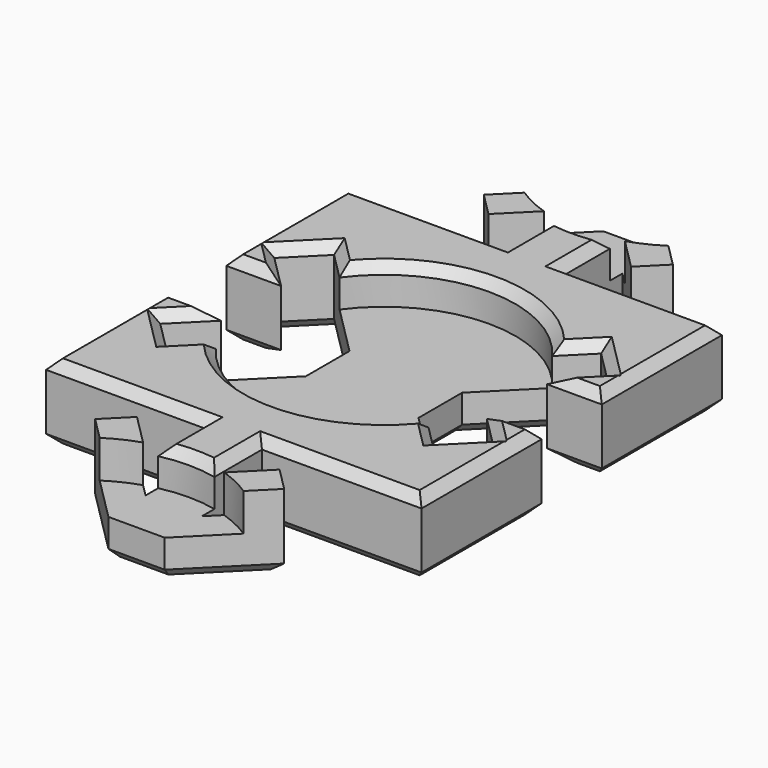
from build123d import *

# Parameters (mm, degrees)
F1_DEPTH      = 4
F4_R          = 7
F5_DEPTH      = 2
F6_T1_DEPTH   = 3.3367062638
F6_T3_DEPTH   = 2.5
F6_T5_DEPTH   = 3.8287347128
F6_T7_DEPTH   = 5.4895762068
F6_T9_DEPTH   = 10.571682988
F6_T11_DEPTH  = 9.785841494
F6_T13_DEPTH  = 4.4484443284
F6_T15_DEPTH  = 9.785841494
F6_T17_DEPTH  = 5.4895762068
F6_T19_DEPTH  = 3.8287347128
F6_T21_DEPTH  = 2.5
F6_T23_DEPTH  = 3.3367062638
F6_T25_DEPTH  = 4.4484443284
F6_T27_DEPTH  = 10.571682988
F6_T29_DEPTH  = 3.8287347128
F6_T31_DEPTH  = 2.5
F6_T33_DEPTH  = 3.3367062638
F6_T35_DEPTH  = 3.3367062638
F6_T37_DEPTH  = 2.5
F6_T39_DEPTH  = 3.8287347128
F6_T41_DEPTH  = 4.321682988
F6_T43_DEPTH  = 4.321682988
F6_T45_DEPTH  = 7.571682988
F6_T47_DEPTH  = 5.571682988
F6_T49_DEPTH  = 7.571682988
F6_T51_DEPTH  = 4.321682988
F6_T53_DEPTH  = 4.321682988
F6_T55_DEPTH  = 7.571682988
F6_T57_DEPTH  = 7.571682988
F6_T60_ANGLE  = 129.037666836
F6_T64_ANGLE  = 45.7974010276
F6_T70_ANGLE  = 45.7974010276
F6_T74_ANGLE  = 129.037666836
F6_T78_DEPTH  = 5.821682988
F6_T83_DEPTH  = 5.285841494
F6_T88_DEPTH  = 7.1017054858
F6_T93_DEPTH  = 5.4785372375
F6_T99_DEPTH  = 7.1017054858
F6_T104_DEPTH = 5.285841494
F6_T109_DEPTH = 5.821682988
F6_T114_DEPTH = 5.821682988
F6_T119_DEPTH = 5.285841494
F6_T124_DEPTH = 7.1017054858
F6_T129_DEPTH = 5.4785372375
F6_T135_DEPTH = 7.1017054858
F6_T140_DEPTH = 5.285841494
F6_T145_DEPTH = 5.821682988
F6_T151_DEPTH = 3.785841494
F6_T155_DEPTH = 4.6225477578
F6_T162_DEPTH = 5.1145762068
F6_T167_DEPTH = 3.785841494
F6_T175_DEPTH = 5.7342858224
F6_T179_DEPTH = 9.785841494
F6_T186_DEPTH = 9.785841494
F6_T190_DEPTH = 5.7342858224
F6_T197_DEPTH = 3.785841494
F6_T202_DEPTH = 5.1145762068
F6_T210_DEPTH = 4.6225477578
F6_T214_DEPTH = 3.785841494
F6_T221_DEPTH = 9.785841494
F6_T225_DEPTH = 5.7342858224
F6_T232_DEPTH = 3.785841494
F6_T237_DEPTH = 5.1145762068
F6_T245_DEPTH = 4.6225477578
F6_T249_DEPTH = 3.785841494
F6_T256_DEPTH = 3.785841494
F6_T260_DEPTH = 4.6225477578
F6_T267_DEPTH = 5.1145762068
F6_T272_DEPTH = 3.785841494
F6_T280_DEPTH = 5.7342858224
F6_T284_DEPTH = 9.785841494
F6_T291_DEPTH = 4.535841494
F6_T295_DEPTH = 5.285841494
F6_T302_DEPTH = 6.571682988
F6_T306_DEPTH = 9.785841494
F6_T313_DEPTH = 5.1145762068
F6_T318_DEPTH = 3.785841494
F6_T326_DEPTH = 3.785841494
F6_T330_DEPTH = 8.3875469798
F6_T337_DEPTH = 7.1017054858
F6_T341_DEPTH = 5.4785372375
F6_T348_DEPTH = 5.4785372375
F6_T352_DEPTH = 7.1017054858
F6_T359_DEPTH = 8.3875469798
F6_T363_DEPTH = 3.785841494
F6_T370_DEPTH = 3.785841494
F6_T375_DEPTH = 5.1145762068
F6_T383_DEPTH = 9.785841494
F6_T387_DEPTH = 6.571682988
F6_T394_DEPTH = 5.285841494
F6_T398_DEPTH = 4.535841494
F6_T405_DEPTH = 4.535841494
F6_T409_DEPTH = 5.285841494
F6_T416_DEPTH = 6.571682988
F6_T420_DEPTH = 9.785841494
F6_T427_DEPTH = 5.1145762068
F6_T432_DEPTH = 3.785841494
F6_T440_DEPTH = 3.785841494
F6_T444_DEPTH = 8.3875469798
F6_T451_DEPTH = 7.1017054858
F6_T455_DEPTH = 5.4785372375
F6_T462_DEPTH = 5.4785372375
F6_T466_DEPTH = 7.1017054858
F6_T473_DEPTH = 8.3875469798
F6_T477_DEPTH = 3.785841494
F6_T484_DEPTH = 3.785841494
F6_T489_DEPTH = 5.1145762068
F6_T497_DEPTH = 9.785841494
F6_T501_DEPTH = 6.571682988
F6_T508_DEPTH = 5.285841494
F6_T512_DEPTH = 4.535841494


# Not quite as in the source:
# - a fillet or chamfer that OpenCascade refuses, or shapes differently, is made with other operations: its cross-section is extruded or revolved along the edge and cut away or added


with BuildPart() as f1:
    # F0 (on Top) → F1 (new body)
    with BuildSketch(Plane.XY):
        Polygon((-1.5, 10), (0, 10), (0, 16.4748737342), (-1.5, 16.4748737342), (-5.0355339059, 12.9393398282), (-3.7980970389, 11.7019029611), (-1.5, 14), align=None)
        Polygon((-3, 0), (0, 0), (0, 10), (-1.5, 10), (-10, 10), (-10, 2), (-7.0821067812, 2), (-8.88020382, 3.7980970389), (-7.1124368671, 5.5658639918), (-3, 1.4534271247), align=None)
    extrude(amount=F1_DEPTH)

    # F2: F1 across plane


with BuildPart() as f1_1:
    add(f1.part)
    add(f1.part.mirror(Plane.YZ))

    # F3: F1 across plane


with BuildPart() as f1_2:
    add(f1_1.part)
    add(f1_1.part.mirror(Plane.XZ))

    # F4 (on face) → F5 (cut)
    with BuildSketch(Plane.XY.offset(4)):
        Circle(F4_R)
        with Locations((0, 20)):
            Circle(F4_R)
        with Locations((0, -20)):
            Circle(F4_R)
    extrude(amount=-F5_DEPTH, mode=Mode.SUBTRACT)

    # F6: chamfer of 0.5 on 76 edges, made by hand

    # F6_s2 → F6_t1 (cut)
    with BuildSketch(Plane(origin=(6.3391504294, -6.3391504294, 0), x_dir=(0, 0, 1), z_dir=(-0.7071067812, 0.7071067812, 0))):
        Polygon((3.5, 1.0935921677), (4, 0.5935921677), (4, 1.0935921677), align=None)
    extrude(amount=F6_T1_DEPTH, mode=Mode.SUBTRACT)

    # F6_s4 → F6_t3 (cut)
    with BuildSketch(Plane(origin=(2.5410533906, 2.5410533906, 0), x_dir=(0, 0, 1), z_dir=(-0.7071067812, -0.7071067812, 0))):
        Polygon((3.5, -8.9649125113), (4, -9.4649125113), (4, -8.9649125113), align=None)
        Polygon((0, -9.4649125113), (0.5, -8.9649125113), (0, -8.9649125113), align=None)
    extrude(amount=F6_T3_DEPTH, mode=Mode.SUBTRACT)

    # F6_s6 → F6_t5 (cut)
    with BuildSketch(Plane(origin=(3.6318261507, -3.6318261507, 0), x_dir=(0, 0, 1), z_dir=(0.7071067812, -0.7071067812, 0))):
        Polygon((3.5, -3.5935921677), (4, -4.0935921677), (4, -3.5935921677), align=None)
        Polygon((0, -4.0935921677), (0.5, -3.5935921677), (0, -3.5935921677), align=None)
    extrude(amount=F6_T5_DEPTH, mode=Mode.SUBTRACT)

    # F6_s8 → F6_t7 (cut)
    with BuildSketch(Plane.YZ.offset(5.7962652872)):
        Polygon((-2, 3.5), (-2.5, 4), (-2, 4), align=None)
        Polygon((2, 3.5), (2.5, 4), (2, 4), align=None)
        Polygon((-2.5, 0), (-2, 0.5), (-2, 0), align=None)
        Polygon((2.5, 0), (2, 0.5), (2, 0), align=None)
    extrude(amount=F6_T7_DEPTH, mode=Mode.SUBTRACT)

    # F6_s10 → F6_t9 (cut)
    with BuildSketch(Plane.XZ.offset(0.714158506)):
        Polygon((10, 3.5), (9.5, 4), (10, 4), align=None)
        Polygon((-10, 3.5), (-9.5, 4), (-10, 4), align=None)
        Polygon((-9.5, 0), (-10, 0.5), (-10, 0), align=None)
        Polygon((9.5, 0), (10, 0.5), (10, 0), align=None)
    extrude(amount=F6_T9_DEPTH, mode=Mode.SUBTRACT)

    # F6_s12 → F6_t11 (cut)
    with BuildSketch(Plane.YZ.offset(1.5)):
        Polygon((-10, 3.5), (-9.5, 4), (-10, 4), align=None)
        Polygon((10, 3.5), (9.5, 4), (10, 4), align=None)
        Polygon((-9.5, 0), (-10, 0.5), (-10, 0), align=None)
        Polygon((9.5, 0), (10, 0.5), (10, 0), align=None)
    extrude(amount=F6_T11_DEPTH, mode=Mode.SUBTRACT)

    # F6_s14 → F6_t13 (cut)
    with BuildSketch(Plane.XZ.offset(10)):
        Polygon((1.5, 3.5), (1, 4), (1.5, 4), align=None)
        Polygon((-1.5, 3.5), (-1, 4), (-1.5, 4), align=None)
    extrude(amount=F6_T13_DEPTH, mode=Mode.SUBTRACT)

    # F6_s16 → F6_t15 (cut)
    with BuildSketch(Plane.YZ.offset(-11.285841494)):
        Polygon((-10, 3.5), (-9.5, 4), (-10, 4), align=None)
        Polygon((10, 3.5), (9.5, 4), (10, 4), align=None)
        Polygon((9.5, 0), (10, 0.5), (10, 0), align=None)
        Polygon((-9.5, 0), (-10, 0.5), (-10, 0), align=None)
    extrude(amount=F6_T15_DEPTH, mode=Mode.SUBTRACT)

    # F6_s18 → F6_t17 (cut)
    with BuildSketch(Plane.YZ.offset(-11.285841494)):
        Polygon((-2, 3.5), (-2.5, 4), (-2, 4), align=None)
        Polygon((2, 3.5), (2.5, 4), (2, 4), align=None)
        Polygon((2.5, 0), (2, 0.5), (2, 0), align=None)
        Polygon((-2.5, 0), (-2, 0.5), (-2, 0), align=None)
    extrude(amount=F6_T17_DEPTH, mode=Mode.SUBTRACT)

    # F6_s20 → F6_t19 (cut)
    with BuildSketch(Plane(origin=(-3.6318261507, -3.6318261507, 0), x_dir=(0, 0, 1), z_dir=(-0.7071067812, -0.7071067812, 0))):
        Polygon((3.5, 3.5935921677), (4, 4.0935921677), (4, 3.5935921677), align=None)
        Polygon((0, 4.0935921677), (0.5, 3.5935921677), (0, 3.5935921677), align=None)
    extrude(amount=F6_T19_DEPTH, mode=Mode.SUBTRACT)

    # F6_s22 → F6_t21 (cut)
    with BuildSketch(Plane(origin=(-2.5410533906, 2.5410533906, 0), x_dir=(0, 0, 1), z_dir=(0.7071067812, -0.7071067812, 0))):
        Polygon((3.5, 8.9649125113), (4, 9.4649125113), (4, 8.9649125113), align=None)
        Polygon((0, 9.4649125113), (0.5, 8.9649125113), (0, 8.9649125113), align=None)
    extrude(amount=F6_T21_DEPTH, mode=Mode.SUBTRACT)

    # F6_s24 → F6_t23 (cut)
    with BuildSketch(Plane(origin=(-6.3391504294, -6.3391504294, 0), x_dir=(0, 0, 1), z_dir=(0.7071067812, 0.7071067812, 0))):
        Polygon((3.5, -1.0935921677), (4, -0.5935921677), (4, -1.0935921677), align=None)
    extrude(amount=F6_T23_DEPTH, mode=Mode.SUBTRACT)

    # F6_s26 → F6_t25 (cut)
    with BuildSketch(Plane.XZ.offset(-14.4484443284)):
        Polygon((1.5, 3.5), (1, 4), (1.5, 4), align=None)
        Polygon((-1.5, 3.5), (-1, 4), (-1.5, 4), align=None)
    extrude(amount=F6_T25_DEPTH, mode=Mode.SUBTRACT)

    # F6_s28 → F6_t27 (cut)
    with BuildSketch(Plane.XZ.offset(-11.285841494)):
        Polygon((10, 3.5), (9.5, 4), (10, 4), align=None)
        Polygon((-10, 3.5), (-9.5, 4), (-10, 4), align=None)
        Polygon((-9.5, 0), (-10, 0.5), (-10, 0), align=None)
        Polygon((9.5, 0), (10, 0.5), (10, 0), align=None)
    extrude(amount=F6_T27_DEPTH, mode=Mode.SUBTRACT)

    # F6_s30 → F6_t29 (cut)
    with BuildSketch(Plane(origin=(3.6318261507, 3.6318261507, 0), x_dir=(0, 0, 1), z_dir=(0.7071067812, 0.7071067812, 0))):
        Polygon((3.5, 3.5935921677), (4, 4.0935921677), (4, 3.5935921677), align=None)
        Polygon((0, 4.0935921677), (0.5, 3.5935921677), (0, 3.5935921677), align=None)
    extrude(amount=F6_T29_DEPTH, mode=Mode.SUBTRACT)

    # F6_s32 → F6_t31 (cut)
    with BuildSketch(Plane(origin=(2.5410533906, -2.5410533906, 0), x_dir=(0, 0, 1), z_dir=(-0.7071067812, 0.7071067812, 0))):
        Polygon((3.5, 8.9649125113), (4, 9.4649125113), (4, 8.9649125113), align=None)
        Polygon((0, 9.4649125113), (0.5, 8.9649125113), (0, 8.9649125113), align=None)
    extrude(amount=F6_T31_DEPTH, mode=Mode.SUBTRACT)

    # F6_s34 → F6_t33 (cut)
    with BuildSketch(Plane(origin=(6.3391504294, 6.3391504294, 0), x_dir=(0, 0, 1), z_dir=(-0.7071067812, -0.7071067812, 0))):
        Polygon((3.5, -1.0935921677), (4, -0.5935921677), (4, -1.0935921677), align=None)
    extrude(amount=F6_T33_DEPTH, mode=Mode.SUBTRACT)

    # F6_s36 → F6_t35 (cut)
    with BuildSketch(Plane(origin=(-6.3391504294, 6.3391504294, 0), x_dir=(0, 0, 1), z_dir=(0.7071067812, -0.7071067812, 0))):
        Polygon((3.5, 1.0935921677), (4, 0.5935921677), (4, 1.0935921677), align=None)
    extrude(amount=F6_T35_DEPTH, mode=Mode.SUBTRACT)

    # F6_s38 → F6_t37 (cut)
    with BuildSketch(Plane(origin=(-2.5410533906, -2.5410533906, 0), x_dir=(0, 0, 1), z_dir=(0.7071067812, 0.7071067812, 0))):
        Polygon((3.5, -8.9649125113), (4, -9.4649125113), (4, -8.9649125113), align=None)
        Polygon((0, -9.4649125113), (0.5, -8.9649125113), (0, -8.9649125113), align=None)
    extrude(amount=F6_T37_DEPTH, mode=Mode.SUBTRACT)

    # F6_s40 → F6_t39 (cut)
    with BuildSketch(Plane(origin=(-3.6318261507, 3.6318261507, 0), x_dir=(0, 0, 1), z_dir=(-0.7071067812, 0.7071067812, 0))):
        Polygon((3.5, -3.5935921677), (4, -4.0935921677), (4, -3.5935921677), align=None)
        Polygon((0, -4.0935921677), (0.5, -3.5935921677), (0, -3.5935921677), align=None)
    extrude(amount=F6_T39_DEPTH, mode=Mode.SUBTRACT)

    # F6_s42 → F6_t41 (cut)
    with BuildSketch(Plane(origin=(-9.896664107, 9.896664107, 0), x_dir=(0, 0, 1), z_dir=(0.7071067812, -0.7071067812, 0))):
        Polygon((0.5, -5.5888347648), (0, -6.0888347648), (0, -5.5888347648), align=None)
    extrude(amount=F6_T41_DEPTH, mode=Mode.SUBTRACT)

    # F6_s44 → F6_t43 (cut)
    with BuildSketch(Plane(origin=(-9.896664107, -9.896664107, 0), x_dir=(0, 0, 1), z_dir=(0.7071067812, 0.7071067812, 0))):
        Polygon((0, 6.0888347648), (0.5, 5.5888347648), (0, 5.5888347648), align=None)
    extrude(amount=F6_T43_DEPTH, mode=Mode.SUBTRACT)

    # F6_s46 → F6_t45 (cut)
    with BuildSketch(Plane(origin=(8.396664107, -8.396664107, 0), x_dir=(0, 0, 1), z_dir=(-0.7071067812, 0.7071067812, 0))):
        Polygon((0, -12.2101551084), (0.5, -12.7101551084), (0, -12.7101551084), align=None)
    extrude(amount=F6_T45_DEPTH, mode=Mode.SUBTRACT)

    # F6_s48 → F6_t47 (cut)
    with BuildSketch(Plane.YZ.offset(-2.785841494)):
        Polygon((-15.9748737342, 0), (-16.4748737342, 0.5), (-16.4748737342, 0), align=None)
        Polygon((15.9748737342, 0), (16.4748737342, 0.5), (16.4748737342, 0), align=None)
    extrude(amount=F6_T47_DEPTH, mode=Mode.SUBTRACT)

    # F6_s50 → F6_t49 (cut)
    with BuildSketch(Plane(origin=(-8.396664107, -8.396664107, 0), x_dir=(0, 0, 1), z_dir=(0.7071067812, 0.7071067812, 0))):
        Polygon((0, 12.2101551084), (0.5, 12.7101551084), (0, 12.7101551084), align=None)
    extrude(amount=F6_T49_DEPTH, mode=Mode.SUBTRACT)

    # F6_s52 → F6_t51 (cut)
    with BuildSketch(Plane(origin=(9.896664107, -9.896664107, 0), x_dir=(0, 0, 1), z_dir=(-0.7071067812, 0.7071067812, 0))):
        Polygon((0, -6.0888347648), (0.5, -5.5888347648), (0, -5.5888347648), align=None)
    extrude(amount=F6_T51_DEPTH, mode=Mode.SUBTRACT)

    # F6_s54 → F6_t53 (cut)
    with BuildSketch(Plane(origin=(9.896664107, 9.896664107, 0), x_dir=(0, 0, 1), z_dir=(-0.7071067812, -0.7071067812, 0))):
        Polygon((0, 6.0888347648), (0.5, 5.5888347648), (0, 5.5888347648), align=None)
    extrude(amount=F6_T53_DEPTH, mode=Mode.SUBTRACT)

    # F6_s56 → F6_t55 (cut)
    with BuildSketch(Plane(origin=(-8.396664107, 8.396664107, 0), x_dir=(0, 0, 1), z_dir=(0.7071067812, -0.7071067812, 0))):
        Polygon((0, -12.2101551084), (0.5, -12.7101551084), (0, -12.7101551084), align=None)
    extrude(amount=F6_T55_DEPTH, mode=Mode.SUBTRACT)

    # F6_s58 → F6_t57 (cut)
    with BuildSketch(Plane(origin=(8.396664107, 8.396664107, 0), x_dir=(0, 0, 1), z_dir=(-0.7071067812, -0.7071067812, 0))):
        Polygon((0.5, 12.7101551084), (0, 12.2101551084), (0, 12.7101551084), align=None)
    extrude(amount=F6_T57_DEPTH, mode=Mode.SUBTRACT)

    # F6_s59 → F6_t60 (revolve, cut)
    with BuildSketch(Plane(origin=(0, 0, 0), x_dir=(0, 0, 1), z_dir=(-0.4302143891, 0.9027267468, 0))):
        Polygon((3.5, -7), (4, -7.5), (4, -7), align=None)
    revolve(axis=Axis((0, 0, 4), (0, 0, 1)), revolution_arc=F6_T60_ANGLE, mode=Mode.SUBTRACT)


with BuildPart() as f6_tool62:
    # F6_s63 → F6_t64 (revolve)
    with BuildSketch(Plane(origin=(7.1687898307, -3.0280237835, 0), x_dir=(0, 0, 1), z_dir=(0.9211942308, -0.3891030573, 0))):
        Polygon((4, 10.9238846156), (3.5, 11.4238846156), (4, 11.4238846156), align=None)
    revolve(axis=Axis((0, -20, 4), (0, 0, 1)), revolution_arc=F6_T64_ANGLE)

    split(bisect_by=Plane(origin=(-7.75, -7.75, 0), x_dir=(0, 0, 1), z_dir=(0.7071067812, 0.7071067812, 0)), keep=Keep.TOP)

    split(bisect_by=Plane.YZ.offset(1.5), keep=Keep.BOTTOM)


with BuildPart() as f1_3:
    add(f1_2.part)

    # F6_t61: cut F6_tool62
    add(f6_tool62.part, mode=Mode.SUBTRACT)


with BuildPart() as f6_tool68:
    # F6_s69 → F6_t70 (revolve)
    with BuildSketch(Plane(origin=(-7.1687898307, 3.0280237835, 0), x_dir=(0, 0, 1), z_dir=(-0.9211942308, 0.3891030573, 0))):
        Polygon((3.5, 11.4238846156), (4, 10.9238846156), (4, 11.4238846156), align=None)
    revolve(axis=Axis((0, 20, 4), (0, 0, 1)), revolution_arc=F6_T70_ANGLE)

    split(bisect_by=Plane.YZ.offset(-1.5), keep=Keep.TOP)

    split(bisect_by=Plane(origin=(7.75, 7.75, 0), x_dir=(0, 0, 1), z_dir=(-0.7071067812, -0.7071067812, 0)), keep=Keep.TOP)


with BuildPart() as f1_4:
    add(f1_3.part)

    # F6_t67: cut F6_tool68
    add(f6_tool68.part, mode=Mode.SUBTRACT)

    # F6_s73 → F6_t74 (revolve, cut)
    with BuildSketch(Plane(origin=(0, 0, 0), x_dir=(0, 0, 1), z_dir=(0.4302143891, -0.9027267468, 0))):
        Polygon((4, -7.5), (3.5, -7), (4, -7), align=None)
    revolve(axis=Axis((0, 0, 4), (0, 0, 1)), revolution_arc=F6_T74_ANGLE, mode=Mode.SUBTRACT)


with BuildPart() as f6_tool76:
    # F6_s77 → F6_t78 (new body)
    with BuildSketch(Plane(origin=(3.0426757212, 3.0426757212, 0), x_dir=(0, 0, 1), z_dir=(0.7071067812, 0.7071067812, 0))):
        Polygon((0.5, -10.9601551084), (0, -11.4601551084), (0, -10.9601551084), align=None)
    extrude(amount=F6_T78_DEPTH)

    split(bisect_by=Plane.YZ.offset(-1.5), keep=Keep.BOTTOM)


with BuildPart() as f1_5:
    add(f1_4.part)

    # F6_t75: cut F6_tool76
    add(f6_tool76.part, mode=Mode.SUBTRACT)


with BuildPart() as f6_tool81:
    # F6_s82 → F6_t83 (new body)
    with BuildSketch(Plane.XZ.offset(-15.285841494)):
        Polygon((-1, 0), (-1.5, 0.5), (-1.5, 0), align=None)
    extrude(amount=F6_T83_DEPTH)

    split(bisect_by=Plane(origin=(-7.75, 7.75, 0), x_dir=(0, 0, 1), z_dir=(0.7071067812, -0.7071067812, 0)), keep=Keep.TOP)


with BuildPart() as f1_6:
    add(f1_5.part)

    # F6_t80: cut F6_tool81
    add(f6_tool81.part, mode=Mode.SUBTRACT)


with BuildPart() as f6_tool86:
    # F6_s87 → F6_t88 (new body)
    with BuildSketch(Plane(origin=(-6.3391504294, 6.3391504294, 0), x_dir=(0, 0, 1), z_dir=(0.7071067812, -0.7071067812, 0))):
        Polygon((0, 0.5935921677), (0.5, 1.0935921677), (0, 1.0935921677), align=None)
    extrude(amount=F6_T88_DEPTH)

    split(bisect_by=Plane.YZ.offset(-3), keep=Keep.BOTTOM)


with BuildPart() as f1_7:
    add(f1_6.part)

    # F6_t85: cut F6_tool86
    add(f6_tool86.part, mode=Mode.SUBTRACT)


with BuildPart() as f6_tool91:
    # F6_s92 → F6_t93 (new body)
    with BuildSketch(Plane.XZ.offset(2.7392686187)):
        Polygon((-2.5, 0), (-3, 0.5), (-3, 0), align=None)
    extrude(amount=-F6_T93_DEPTH)

    split(bisect_by=Plane(origin=(-0.7732864376, -0.7732864376, 0), x_dir=(0, 0, 1), z_dir=(-0.7071067812, -0.7071067812, 0)), keep=Keep.TOP)

    split(bisect_by=Plane(origin=(-0.7732864376, 0.7732864376, 0), x_dir=(0, 0, 1), z_dir=(-0.7071067812, 0.7071067812, 0)), keep=Keep.TOP)


with BuildPart() as f1_8:
    add(f1_7.part)

    # F6_t90: cut F6_tool91
    add(f6_tool91.part, mode=Mode.SUBTRACT)


with BuildPart() as f6_tool97:
    # F6_s98 → F6_t99 (new body)
    with BuildSketch(Plane(origin=(-6.3391504294, -6.3391504294, 0), x_dir=(0, 0, 1), z_dir=(0.7071067812, 0.7071067812, 0))):
        Polygon((0, -0.5935921677), (0.5, -1.0935921677), (0, -1.0935921677), align=None)
    extrude(amount=F6_T99_DEPTH)

    split(bisect_by=Plane.YZ.offset(-3), keep=Keep.BOTTOM)


with BuildPart() as f1_9:
    add(f1_8.part)

    # F6_t96: cut F6_tool97
    add(f6_tool97.part, mode=Mode.SUBTRACT)


with BuildPart() as f6_tool102:
    # F6_s103 → F6_t104 (new body)
    with BuildSketch(Plane.XZ.offset(15.285841494)):
        Polygon((-1, 0), (-1.5, 0.5), (-1.5, 0), align=None)
    extrude(amount=-F6_T104_DEPTH)

    split(bisect_by=Plane(origin=(-7.75, -7.75, 0), x_dir=(0, 0, 1), z_dir=(0.7071067812, 0.7071067812, 0)), keep=Keep.TOP)


with BuildPart() as f1_10:
    add(f1_9.part)

    # F6_t101: cut F6_tool102
    add(f6_tool102.part, mode=Mode.SUBTRACT)


with BuildPart() as f6_tool107:
    # F6_s108 → F6_t109 (new body)
    with BuildSketch(Plane(origin=(3.0426757212, -3.0426757212, 0), x_dir=(0, 0, 1), z_dir=(0.7071067812, -0.7071067812, 0))):
        Polygon((0, 11.4601551084), (0.5, 10.9601551084), (0, 10.9601551084), align=None)
    extrude(amount=F6_T109_DEPTH)

    split(bisect_by=Plane.YZ.offset(-1.5), keep=Keep.BOTTOM)


with BuildPart() as f1_11:
    add(f1_10.part)

    # F6_t106: cut F6_tool107
    add(f6_tool107.part, mode=Mode.SUBTRACT)


with BuildPart() as f6_tool112:
    # F6_s113 → F6_t114 (new body)
    with BuildSketch(Plane(origin=(-3.0426757212, -3.0426757212, 0), x_dir=(0, 0, 1), z_dir=(-0.7071067812, -0.7071067812, 0))):
        Polygon((0, -11.4601551084), (0.5, -10.9601551084), (0, -10.9601551084), align=None)
    extrude(amount=F6_T114_DEPTH)

    split(bisect_by=Plane.YZ.offset(1.5), keep=Keep.TOP)


with BuildPart() as f1_12:
    add(f1_11.part)

    # F6_t111: cut F6_tool112
    add(f6_tool112.part, mode=Mode.SUBTRACT)


with BuildPart() as f6_tool117:
    # F6_s118 → F6_t119 (new body)
    with BuildSketch(Plane.XZ.offset(15.285841494)):
        Polygon((1, 0), (1.5, 0.5), (1.5, 0), align=None)
    extrude(amount=-F6_T119_DEPTH)

    split(bisect_by=Plane(origin=(7.75, -7.75, 0), x_dir=(0, 0, 1), z_dir=(-0.7071067812, 0.7071067812, 0)), keep=Keep.TOP)


with BuildPart() as f1_13:
    add(f1_12.part)

    # F6_t116: cut F6_tool117
    add(f6_tool117.part, mode=Mode.SUBTRACT)


with BuildPart() as f6_tool122:
    # F6_s123 → F6_t124 (new body)
    with BuildSketch(Plane(origin=(6.3391504294, -6.3391504294, 0), x_dir=(0, 0, 1), z_dir=(-0.7071067812, 0.7071067812, 0))):
        Polygon((0, 0.5935921677), (0.5, 1.0935921677), (0, 1.0935921677), align=None)
    extrude(amount=F6_T124_DEPTH)

    split(bisect_by=Plane.YZ.offset(3), keep=Keep.TOP)


with BuildPart() as f1_14:
    add(f1_13.part)

    # F6_t121: cut F6_tool122
    add(f6_tool122.part, mode=Mode.SUBTRACT)


with BuildPart() as f6_tool127:
    # F6_s128 → F6_t129 (new body)
    with BuildSketch(Plane.XZ.offset(-2.7392686187)):
        Polygon((2.5, 0), (3, 0.5), (3, 0), align=None)
    extrude(amount=F6_T129_DEPTH)

    split(bisect_by=Plane(origin=(0.7732864376, 0.7732864376, 0), x_dir=(0, 0, 1), z_dir=(0.7071067812, 0.7071067812, 0)), keep=Keep.TOP)

    split(bisect_by=Plane(origin=(0.7732864376, -0.7732864376, 0), x_dir=(0, 0, 1), z_dir=(0.7071067812, -0.7071067812, 0)), keep=Keep.TOP)


with BuildPart() as f1_15:
    add(f1_14.part)

    # F6_t126: cut F6_tool127
    add(f6_tool127.part, mode=Mode.SUBTRACT)


with BuildPart() as f6_tool133:
    # F6_s134 → F6_t135 (new body)
    with BuildSketch(Plane(origin=(6.3391504294, 6.3391504294, 0), x_dir=(0, 0, 1), z_dir=(-0.7071067812, -0.7071067812, 0))):
        Polygon((0, -0.5935921677), (0.5, -1.0935921677), (0, -1.0935921677), align=None)
    extrude(amount=F6_T135_DEPTH)

    split(bisect_by=Plane.YZ.offset(3), keep=Keep.TOP)


with BuildPart() as f1_16:
    add(f1_15.part)

    # F6_t132: cut F6_tool133
    add(f6_tool133.part, mode=Mode.SUBTRACT)


with BuildPart() as f6_tool138:
    # F6_s139 → F6_t140 (new body)
    with BuildSketch(Plane.XZ.offset(-15.285841494)):
        Polygon((1, 0), (1.5, 0.5), (1.5, 0), align=None)
    extrude(amount=F6_T140_DEPTH)

    split(bisect_by=Plane(origin=(7.75, 7.75, 0), x_dir=(0, 0, 1), z_dir=(-0.7071067812, -0.7071067812, 0)), keep=Keep.TOP)


with BuildPart() as f1_17:
    add(f1_16.part)

    # F6_t137: cut F6_tool138
    add(f6_tool138.part, mode=Mode.SUBTRACT)


with BuildPart() as f6_tool143:
    # F6_s144 → F6_t145 (new body)
    with BuildSketch(Plane(origin=(-3.0426757212, 3.0426757212, 0), x_dir=(0, 0, 1), z_dir=(-0.7071067812, 0.7071067812, 0))):
        Polygon((0, 11.4601551084), (0.5, 10.9601551084), (0, 10.9601551084), align=None)
    extrude(amount=F6_T145_DEPTH)

    split(bisect_by=Plane.YZ.offset(1.5), keep=Keep.TOP)


with BuildPart() as f1_18:
    add(f1_17.part)

    # F6_t142: cut F6_tool143
    add(f6_tool143.part, mode=Mode.SUBTRACT)


with BuildPart() as f6_tool149:
    # F6_s150 → F6_t151 (new body)
    with BuildSketch(Plane(origin=(2.5410533906, 2.5410533906, 0), x_dir=(0, 0, 1), z_dir=(-0.7071067812, -0.7071067812, 0))):
        Polygon((3.5, -8.9649125113), (4, -9.4649125113), (4, -8.9649125113), align=None)
    extrude(amount=F6_T151_DEPTH)

    split(bisect_by=Plane(origin=(0.7732864376, 0.7732864376, 0), x_dir=(0, 0, 1), z_dir=(-0.7071067812, -0.7071067812, 0)), keep=Keep.TOP)


with BuildPart() as f6_tool153:
    # F6_s154 → F6_t155 (new body)
    with BuildSketch(Plane(origin=(7.2483776694, -7.2483776694, 0), x_dir=(0, 0, 1), z_dir=(-0.7071067812, 0.7071067812, 0))):
        Polygon((3.5, 1.0935921677), (4, 0.5935921677), (4, 1.0935921677), align=None)
    extrude(amount=F6_T155_DEPTH)

    split(bisect_by=Plane(origin=(6.3391504294, -6.3391504294, 0), x_dir=(0, 0, 1), z_dir=(0.7071067812, -0.7071067812, 0)), keep=Keep.TOP)


with BuildPart() as f6_tool149_1:
    add(f6_tool149.part)

    # F6_t157: intersect F6_tool153
    add(f6_tool153.part, mode=Mode.INTERSECT)


with BuildPart() as f1_19:
    add(f1_18.part)

    # F6_t147: cut F6_tool149
    add(f6_tool149_1.part, mode=Mode.SUBTRACT)


with BuildPart() as f6_tool160:
    # F6_s161 → F6_t162 (new body)
    with BuildSketch(Plane(origin=(3.6318261507, -3.6318261507, 0), x_dir=(0, 0, 1), z_dir=(0.7071067812, -0.7071067812, 0))):
        Polygon((3.5, -3.5935921677), (4, -4.0935921677), (4, -3.5935921677), align=None)
    extrude(amount=F6_T162_DEPTH)

    split(bisect_by=Plane.YZ.offset(10), keep=Keep.BOTTOM)

    split(bisect_by=Plane(origin=(6.3391504294, -6.3391504294, 0), x_dir=(0, 0, 1), z_dir=(0.7071067812, -0.7071067812, 0)), keep=Keep.TOP)


with BuildPart() as f6_tool165:
    # F6_s166 → F6_t167 (new body)
    with BuildSketch(Plane(origin=(3.4502806305, 3.4502806305, 0), x_dir=(0, 0, 1), z_dir=(-0.7071067812, -0.7071067812, 0))):
        Polygon((3.5, -8.9649125113), (4, -9.4649125113), (4, -8.9649125113), align=None)
    extrude(amount=F6_T167_DEPTH)

    split(bisect_by=Plane.YZ.offset(10), keep=Keep.BOTTOM)

    split(bisect_by=Plane(origin=(2.5410533906, 2.5410533906, 0), x_dir=(0, 0, 1), z_dir=(0.7071067812, 0.7071067812, 0)), keep=Keep.TOP)


with BuildPart() as f6_tool160_1:
    add(f6_tool160.part)

    # F6_t170: intersect F6_tool165
    add(f6_tool165.part, mode=Mode.INTERSECT)


with BuildPart() as f1_20:
    add(f1_19.part)

    # F6_t158: cut F6_tool160
    add(f6_tool160_1.part, mode=Mode.SUBTRACT)


with BuildPart() as f6_tool173:
    # F6_s174 → F6_t175 (new body)
    with BuildSketch(Plane.XZ.offset(14.4484443284)):
        Polygon((1.5, 3.5), (1, 4), (1.5, 4), align=None)
    extrude(amount=-F6_T175_DEPTH)

    split(bisect_by=Plane.XZ.offset(10), keep=Keep.BOTTOM)


with BuildPart() as f6_tool177:
    # F6_s178 → F6_t179 (new body)
    with BuildSketch(Plane.YZ.offset(0.214158506)):
        Polygon((-10, 3.5), (-9.5, 4), (-10, 4), align=None)
    extrude(amount=F6_T179_DEPTH)

    split(bisect_by=Plane.YZ.offset(1.5), keep=Keep.BOTTOM)


with BuildPart() as f6_tool173_1:
    add(f6_tool173.part)

    # F6_t181: intersect F6_tool177
    add(f6_tool177.part, mode=Mode.INTERSECT)


with BuildPart() as f1_21:
    add(f1_20.part)

    # F6_t171: cut F6_tool173
    add(f6_tool173_1.part, mode=Mode.SUBTRACT)


with BuildPart() as f6_tool184:
    # F6_s185 → F6_t186 (new body)
    with BuildSketch(Plane.YZ.offset(-0.214158506)):
        Polygon((-10, 3.5), (-9.5, 4), (-10, 4), align=None)
    extrude(amount=-F6_T186_DEPTH)

    split(bisect_by=Plane.YZ.offset(-1.5), keep=Keep.TOP)


with BuildPart() as f6_tool188:
    # F6_s189 → F6_t190 (new body)
    with BuildSketch(Plane.XZ.offset(14.4484443284)):
        Polygon((-1.5, 3.5), (-1, 4), (-1.5, 4), align=None)
    extrude(amount=-F6_T190_DEPTH)

    split(bisect_by=Plane.XZ.offset(10), keep=Keep.BOTTOM)


with BuildPart() as f6_tool184_1:
    add(f6_tool184.part)

    # F6_t192: intersect F6_tool188
    add(f6_tool188.part, mode=Mode.INTERSECT)


with BuildPart() as f1_22:
    add(f1_21.part)

    # F6_t182: cut F6_tool184
    add(f6_tool184_1.part, mode=Mode.SUBTRACT)


with BuildPart() as f6_tool195:
    # F6_s196 → F6_t197 (new body)
    with BuildSketch(Plane(origin=(-3.4502806305, 3.4502806305, 0), x_dir=(0, 0, 1), z_dir=(0.7071067812, -0.7071067812, 0))):
        Polygon((3.5, 8.9649125113), (4, 9.4649125113), (4, 8.9649125113), align=None)
    extrude(amount=F6_T197_DEPTH)

    split(bisect_by=Plane(origin=(-2.5410533906, 2.5410533906, 0), x_dir=(0, 0, 1), z_dir=(-0.7071067812, 0.7071067812, 0)), keep=Keep.TOP)

    split(bisect_by=Plane.YZ.offset(-10), keep=Keep.TOP)


with BuildPart() as f6_tool200:
    # F6_s201 → F6_t202 (new body)
    with BuildSketch(Plane(origin=(-3.6318261507, -3.6318261507, 0), x_dir=(0, 0, 1), z_dir=(-0.7071067812, -0.7071067812, 0))):
        Polygon((3.5, 3.5935921677), (4, 4.0935921677), (4, 3.5935921677), align=None)
    extrude(amount=F6_T202_DEPTH)

    split(bisect_by=Plane(origin=(-6.3391504294, -6.3391504294, 0), x_dir=(0, 0, 1), z_dir=(-0.7071067812, -0.7071067812, 0)), keep=Keep.TOP)

    split(bisect_by=Plane.YZ.offset(-10), keep=Keep.TOP)


with BuildPart() as f6_tool195_1:
    add(f6_tool195.part)

    # F6_t205: intersect F6_tool200
    add(f6_tool200.part, mode=Mode.INTERSECT)


with BuildPart() as f1_23:
    add(f1_22.part)

    # F6_t193: cut F6_tool195
    add(f6_tool195_1.part, mode=Mode.SUBTRACT)


with BuildPart() as f6_tool208:
    # F6_s209 → F6_t210 (new body)
    with BuildSketch(Plane(origin=(-7.2483776694, -7.2483776694, 0), x_dir=(0, 0, 1), z_dir=(0.7071067812, 0.7071067812, 0))):
        Polygon((3.5, -1.0935921677), (4, -0.5935921677), (4, -1.0935921677), align=None)
    extrude(amount=F6_T210_DEPTH)

    split(bisect_by=Plane(origin=(-6.3391504294, -6.3391504294, 0), x_dir=(0, 0, 1), z_dir=(-0.7071067812, -0.7071067812, 0)), keep=Keep.TOP)


with BuildPart() as f6_tool212:
    # F6_s213 → F6_t214 (new body)
    with BuildSketch(Plane(origin=(-2.5410533906, 2.5410533906, 0), x_dir=(0, 0, 1), z_dir=(0.7071067812, -0.7071067812, 0))):
        Polygon((3.5, 8.9649125113), (4, 9.4649125113), (4, 8.9649125113), align=None)
    extrude(amount=F6_T214_DEPTH)

    split(bisect_by=Plane(origin=(-0.7732864376, 0.7732864376, 0), x_dir=(0, 0, 1), z_dir=(0.7071067812, -0.7071067812, 0)), keep=Keep.TOP)


with BuildPart() as f6_tool208_1:
    add(f6_tool208.part)

    # F6_t216: intersect F6_tool212
    add(f6_tool212.part, mode=Mode.INTERSECT)


with BuildPart() as f1_24:
    add(f1_23.part)

    # F6_t206: cut F6_tool208
    add(f6_tool208_1.part, mode=Mode.SUBTRACT)


with BuildPart() as f6_tool219:
    # F6_s220 → F6_t221 (new body)
    with BuildSketch(Plane.YZ.offset(0.214158506)):
        Polygon((10, 3.5), (9.5, 4), (10, 4), align=None)
    extrude(amount=F6_T221_DEPTH)

    split(bisect_by=Plane.YZ.offset(1.5), keep=Keep.BOTTOM)


with BuildPart() as f6_tool223:
    # F6_s224 → F6_t225 (new body)
    with BuildSketch(Plane.XZ.offset(-14.4484443284)):
        Polygon((1.5, 3.5), (1, 4), (1.5, 4), align=None)
    extrude(amount=F6_T225_DEPTH)

    split(bisect_by=Plane.XZ.offset(-10), keep=Keep.TOP)


with BuildPart() as f6_tool219_1:
    add(f6_tool219.part)

    # F6_t227: intersect F6_tool223
    add(f6_tool223.part, mode=Mode.INTERSECT)


with BuildPart() as f1_25:
    add(f1_24.part)

    # F6_t217: cut F6_tool219
    add(f6_tool219_1.part, mode=Mode.SUBTRACT)


with BuildPart() as f6_tool230:
    # F6_s231 → F6_t232 (new body)
    with BuildSketch(Plane(origin=(3.4502806305, -3.4502806305, 0), x_dir=(0, 0, 1), z_dir=(-0.7071067812, 0.7071067812, 0))):
        Polygon((3.5, 8.9649125113), (4, 9.4649125113), (4, 8.9649125113), align=None)
    extrude(amount=F6_T232_DEPTH)

    split(bisect_by=Plane(origin=(2.5410533906, -2.5410533906, 0), x_dir=(0, 0, 1), z_dir=(0.7071067812, -0.7071067812, 0)), keep=Keep.TOP)

    split(bisect_by=Plane.YZ.offset(10), keep=Keep.BOTTOM)


with BuildPart() as f6_tool235:
    # F6_s236 → F6_t237 (new body)
    with BuildSketch(Plane(origin=(3.6318261507, 3.6318261507, 0), x_dir=(0, 0, 1), z_dir=(0.7071067812, 0.7071067812, 0))):
        Polygon((3.5, 3.5935921677), (4, 4.0935921677), (4, 3.5935921677), align=None)
    extrude(amount=F6_T237_DEPTH)

    split(bisect_by=Plane(origin=(6.3391504294, 6.3391504294, 0), x_dir=(0, 0, 1), z_dir=(0.7071067812, 0.7071067812, 0)), keep=Keep.TOP)

    split(bisect_by=Plane.YZ.offset(10), keep=Keep.BOTTOM)


with BuildPart() as f6_tool230_1:
    add(f6_tool230.part)

    # F6_t240: intersect F6_tool235
    add(f6_tool235.part, mode=Mode.INTERSECT)


with BuildPart() as f1_26:
    add(f1_25.part)

    # F6_t228: cut F6_tool230
    add(f6_tool230_1.part, mode=Mode.SUBTRACT)


with BuildPart() as f6_tool243:
    # F6_s244 → F6_t245 (new body)
    with BuildSketch(Plane(origin=(7.2483776694, 7.2483776694, 0), x_dir=(0, 0, 1), z_dir=(-0.7071067812, -0.7071067812, 0))):
        Polygon((3.5, -1.0935921677), (4, -0.5935921677), (4, -1.0935921677), align=None)
    extrude(amount=F6_T245_DEPTH)

    split(bisect_by=Plane(origin=(6.3391504294, 6.3391504294, 0), x_dir=(0, 0, 1), z_dir=(0.7071067812, 0.7071067812, 0)), keep=Keep.TOP)


with BuildPart() as f6_tool247:
    # F6_s248 → F6_t249 (new body)
    with BuildSketch(Plane(origin=(2.5410533906, -2.5410533906, 0), x_dir=(0, 0, 1), z_dir=(-0.7071067812, 0.7071067812, 0))):
        Polygon((3.5, 8.9649125113), (4, 9.4649125113), (4, 8.9649125113), align=None)
    extrude(amount=F6_T249_DEPTH)

    split(bisect_by=Plane(origin=(0.7732864376, -0.7732864376, 0), x_dir=(0, 0, 1), z_dir=(-0.7071067812, 0.7071067812, 0)), keep=Keep.TOP)


with BuildPart() as f6_tool243_1:
    add(f6_tool243.part)

    # F6_t251: intersect F6_tool247
    add(f6_tool247.part, mode=Mode.INTERSECT)


with BuildPart() as f1_27:
    add(f1_26.part)

    # F6_t241: cut F6_tool243
    add(f6_tool243_1.part, mode=Mode.SUBTRACT)


with BuildPart() as f6_tool254:
    # F6_s255 → F6_t256 (new body)
    with BuildSketch(Plane(origin=(-2.5410533906, -2.5410533906, 0), x_dir=(0, 0, 1), z_dir=(0.7071067812, 0.7071067812, 0))):
        Polygon((3.5, -8.9649125113), (4, -9.4649125113), (4, -8.9649125113), align=None)
    extrude(amount=F6_T256_DEPTH)

    split(bisect_by=Plane(origin=(-0.7732864376, -0.7732864376, 0), x_dir=(0, 0, 1), z_dir=(0.7071067812, 0.7071067812, 0)), keep=Keep.TOP)


with BuildPart() as f6_tool258:
    # F6_s259 → F6_t260 (new body)
    with BuildSketch(Plane(origin=(-7.2483776694, 7.2483776694, 0), x_dir=(0, 0, 1), z_dir=(0.7071067812, -0.7071067812, 0))):
        Polygon((3.5, 1.0935921677), (4, 0.5935921677), (4, 1.0935921677), align=None)
    extrude(amount=F6_T260_DEPTH)

    split(bisect_by=Plane(origin=(-6.3391504294, 6.3391504294, 0), x_dir=(0, 0, 1), z_dir=(-0.7071067812, 0.7071067812, 0)), keep=Keep.TOP)


with BuildPart() as f6_tool254_1:
    add(f6_tool254.part)

    # F6_t262: intersect F6_tool258
    add(f6_tool258.part, mode=Mode.INTERSECT)


with BuildPart() as f1_28:
    add(f1_27.part)

    # F6_t252: cut F6_tool254
    add(f6_tool254_1.part, mode=Mode.SUBTRACT)


with BuildPart() as f6_tool265:
    # F6_s266 → F6_t267 (new body)
    with BuildSketch(Plane(origin=(-3.6318261507, 3.6318261507, 0), x_dir=(0, 0, 1), z_dir=(-0.7071067812, 0.7071067812, 0))):
        Polygon((3.5, -3.5935921677), (4, -4.0935921677), (4, -3.5935921677), align=None)
    extrude(amount=F6_T267_DEPTH)

    split(bisect_by=Plane.YZ.offset(-10), keep=Keep.TOP)

    split(bisect_by=Plane(origin=(-6.3391504294, 6.3391504294, 0), x_dir=(0, 0, 1), z_dir=(-0.7071067812, 0.7071067812, 0)), keep=Keep.TOP)


with BuildPart() as f6_tool270:
    # F6_s271 → F6_t272 (new body)
    with BuildSketch(Plane(origin=(-3.4502806305, -3.4502806305, 0), x_dir=(0, 0, 1), z_dir=(0.7071067812, 0.7071067812, 0))):
        Polygon((3.5, -8.9649125113), (4, -9.4649125113), (4, -8.9649125113), align=None)
    extrude(amount=F6_T272_DEPTH)

    split(bisect_by=Plane.YZ.offset(-10), keep=Keep.TOP)

    split(bisect_by=Plane(origin=(-2.5410533906, -2.5410533906, 0), x_dir=(0, 0, 1), z_dir=(-0.7071067812, -0.7071067812, 0)), keep=Keep.TOP)


with BuildPart() as f6_tool265_1:
    add(f6_tool265.part)

    # F6_t275: intersect F6_tool270
    add(f6_tool270.part, mode=Mode.INTERSECT)


with BuildPart() as f1_29:
    add(f1_28.part)

    # F6_t263: cut F6_tool265
    add(f6_tool265_1.part, mode=Mode.SUBTRACT)


with BuildPart() as f6_tool278:
    # F6_s279 → F6_t280 (new body)
    with BuildSketch(Plane.XZ.offset(-14.4484443284)):
        Polygon((-1.5, 3.5), (-1, 4), (-1.5, 4), align=None)
    extrude(amount=F6_T280_DEPTH)

    split(bisect_by=Plane.XZ.offset(-10), keep=Keep.TOP)


with BuildPart() as f6_tool282:
    # F6_s283 → F6_t284 (new body)
    with BuildSketch(Plane.YZ.offset(-0.214158506)):
        Polygon((10, 3.5), (9.5, 4), (10, 4), align=None)
    extrude(amount=-F6_T284_DEPTH)

    split(bisect_by=Plane.YZ.offset(-1.5), keep=Keep.TOP)


with BuildPart() as f6_tool278_1:
    add(f6_tool278.part)

    # F6_t286: intersect F6_tool282
    add(f6_tool282.part, mode=Mode.INTERSECT)


with BuildPart() as f1_30:
    add(f1_29.part)

    # F6_t276: cut F6_tool278
    add(f6_tool278_1.part, mode=Mode.SUBTRACT)


with BuildPart() as f6_tool289:
    # F6_s290 → F6_t291 (new body)
    with BuildSketch(Plane(origin=(3.9519029611, 3.9519029611, 0), x_dir=(0, 0, 1), z_dir=(0.7071067812, 0.7071067812, 0))):
        Polygon((0.5, -10.9601551084), (0, -11.4601551084), (0, -10.9601551084), align=None)
    extrude(amount=F6_T291_DEPTH)

    split(bisect_by=Plane.YZ.offset(-1.5), keep=Keep.TOP)


with BuildPart() as f6_tool293:
    # F6_s294 → F6_t295 (new body)
    with BuildSketch(Plane.XZ.offset(-15.285841494)):
        Polygon((-1, 0), (-1.5, 0.5), (-1.5, 0), align=None)
    extrude(amount=F6_T295_DEPTH)

    split(bisect_by=Plane(origin=(-7.75, 7.75, 0), x_dir=(0, 0, 1), z_dir=(-0.7071067812, 0.7071067812, 0)), keep=Keep.TOP)


with BuildPart() as f6_tool289_1:
    add(f6_tool289.part)

    # F6_t297: intersect F6_tool293
    add(f6_tool293.part, mode=Mode.INTERSECT)


with BuildPart() as f1_31:
    add(f1_30.part)

    # F6_t287: cut F6_tool289
    add(f6_tool289_1.part, mode=Mode.SUBTRACT)


with BuildPart() as f6_tool300:
    # F6_s301 → F6_t302 (new body)
    with BuildSketch(Plane.XZ.offset(-15.285841494)):
        Polygon((-1, 0), (-1.5, 0.5), (-1.5, 0), align=None)
    extrude(amount=F6_T302_DEPTH)

    split(bisect_by=Plane.XZ.offset(-10), keep=Keep.TOP)


with BuildPart() as f6_tool304:
    # F6_s305 → F6_t306 (new body)
    with BuildSketch(Plane.YZ.offset(-0.214158506)):
        Polygon((9.5, 0), (10, 0.5), (10, 0), align=None)
    extrude(amount=-F6_T306_DEPTH)

    split(bisect_by=Plane.YZ.offset(-1.5), keep=Keep.TOP)


with BuildPart() as f6_tool300_1:
    add(f6_tool300.part)

    # F6_t308: intersect F6_tool304
    add(f6_tool304.part, mode=Mode.INTERSECT)


with BuildPart() as f1_32:
    add(f1_31.part)

    # F6_t298: cut F6_tool300
    add(f6_tool300_1.part, mode=Mode.SUBTRACT)


with BuildPart() as f6_tool311:
    # F6_s312 → F6_t313 (new body)
    with BuildSketch(Plane(origin=(-3.6318261507, 3.6318261507, 0), x_dir=(0, 0, 1), z_dir=(-0.7071067812, 0.7071067812, 0))):
        Polygon((0, -4.0935921677), (0.5, -3.5935921677), (0, -3.5935921677), align=None)
    extrude(amount=F6_T313_DEPTH)

    split(bisect_by=Plane.YZ.offset(-10), keep=Keep.TOP)

    split(bisect_by=Plane(origin=(-6.3391504294, 6.3391504294, 0), x_dir=(0, 0, 1), z_dir=(-0.7071067812, 0.7071067812, 0)), keep=Keep.TOP)


with BuildPart() as f6_tool316:
    # F6_s317 → F6_t318 (new body)
    with BuildSketch(Plane(origin=(-3.4502806305, -3.4502806305, 0), x_dir=(0, 0, 1), z_dir=(0.7071067812, 0.7071067812, 0))):
        Polygon((0, -9.4649125113), (0.5, -8.9649125113), (0, -8.9649125113), align=None)
    extrude(amount=F6_T318_DEPTH)

    split(bisect_by=Plane.YZ.offset(-10), keep=Keep.TOP)

    split(bisect_by=Plane(origin=(-2.5410533906, -2.5410533906, 0), x_dir=(0, 0, 1), z_dir=(-0.7071067812, -0.7071067812, 0)), keep=Keep.TOP)


with BuildPart() as f6_tool311_1:
    add(f6_tool311.part)

    # F6_t321: intersect F6_tool316
    add(f6_tool316.part, mode=Mode.INTERSECT)


with BuildPart() as f1_33:
    add(f1_32.part)

    # F6_t309: cut F6_tool311
    add(f6_tool311_1.part, mode=Mode.SUBTRACT)


with BuildPart() as f6_tool324:
    # F6_s325 → F6_t326 (new body)
    with BuildSketch(Plane(origin=(-2.5410533906, -2.5410533906, 0), x_dir=(0, 0, 1), z_dir=(0.7071067812, 0.7071067812, 0))):
        Polygon((0, -9.4649125113), (0.5, -8.9649125113), (0, -8.9649125113), align=None)
    extrude(amount=F6_T326_DEPTH)

    split(bisect_by=Plane(origin=(-0.7732864376, -0.7732864376, 0), x_dir=(0, 0, 1), z_dir=(0.7071067812, 0.7071067812, 0)), keep=Keep.TOP)


with BuildPart() as f6_tool328:
    # F6_s329 → F6_t330 (new body)
    with BuildSketch(Plane(origin=(-7.2483776694, 7.2483776694, 0), x_dir=(0, 0, 1), z_dir=(0.7071067812, -0.7071067812, 0))):
        Polygon((0, 0.5935921677), (0.5, 1.0935921677), (0, 1.0935921677), align=None)
    extrude(amount=F6_T330_DEPTH)

    split(bisect_by=Plane(origin=(-6.3391504294, 6.3391504294, 0), x_dir=(0, 0, 1), z_dir=(-0.7071067812, 0.7071067812, 0)), keep=Keep.TOP)


with BuildPart() as f6_tool324_1:
    add(f6_tool324.part)

    # F6_t332: intersect F6_tool328
    add(f6_tool328.part, mode=Mode.INTERSECT)


with BuildPart() as f1_34:
    add(f1_33.part)

    # F6_t322: cut F6_tool324
    add(f6_tool324_1.part, mode=Mode.SUBTRACT)


with BuildPart() as f6_tool335:
    # F6_s336 → F6_t337 (new body)
    with BuildSketch(Plane(origin=(-6.3391504294, 6.3391504294, 0), x_dir=(0, 0, 1), z_dir=(0.7071067812, -0.7071067812, 0))):
        Polygon((0, 0.5935921677), (0.5, 1.0935921677), (0, 1.0935921677), align=None)
    extrude(amount=F6_T337_DEPTH)

    split(bisect_by=Plane.YZ.offset(-3), keep=Keep.TOP)


with BuildPart() as f6_tool339:
    # F6_s340 → F6_t341 (new body)
    with BuildSketch(Plane.XZ.offset(2.7392686187)):
        Polygon((-2.5, 0), (-3, 0.5), (-3, 0), align=None)
    extrude(amount=-F6_T341_DEPTH)

    split(bisect_by=Plane(origin=(-0.7732864376, -0.7732864376, 0), x_dir=(0, 0, 1), z_dir=(0.7071067812, 0.7071067812, 0)), keep=Keep.TOP)


with BuildPart() as f6_tool335_1:
    add(f6_tool335.part)

    # F6_t343: intersect F6_tool339
    add(f6_tool339.part, mode=Mode.INTERSECT)


with BuildPart() as f1_35:
    add(f1_34.part)

    # F6_t333: cut F6_tool335
    add(f6_tool335_1.part, mode=Mode.SUBTRACT)


with BuildPart() as f6_tool346:
    # F6_s347 → F6_t348 (new body)
    with BuildSketch(Plane.XZ.offset(2.7392686187)):
        Polygon((-2.5, 0), (-3, 0.5), (-3, 0), align=None)
    extrude(amount=-F6_T348_DEPTH)

    split(bisect_by=Plane(origin=(-0.7732864376, 0.7732864376, 0), x_dir=(0, 0, 1), z_dir=(0.7071067812, -0.7071067812, 0)), keep=Keep.TOP)


with BuildPart() as f6_tool350:
    # F6_s351 → F6_t352 (new body)
    with BuildSketch(Plane(origin=(-6.3391504294, -6.3391504294, 0), x_dir=(0, 0, 1), z_dir=(0.7071067812, 0.7071067812, 0))):
        Polygon((0, -0.5935921677), (0.5, -1.0935921677), (0, -1.0935921677), align=None)
    extrude(amount=F6_T352_DEPTH)

    split(bisect_by=Plane.YZ.offset(-3), keep=Keep.TOP)


with BuildPart() as f6_tool346_1:
    add(f6_tool346.part)

    # F6_t354: intersect F6_tool350
    add(f6_tool350.part, mode=Mode.INTERSECT)


with BuildPart() as f1_36:
    add(f1_35.part)

    # F6_t344: cut F6_tool346
    add(f6_tool346_1.part, mode=Mode.SUBTRACT)


with BuildPart() as f6_tool357:
    # F6_s358 → F6_t359 (new body)
    with BuildSketch(Plane(origin=(-7.2483776694, -7.2483776694, 0), x_dir=(0, 0, 1), z_dir=(0.7071067812, 0.7071067812, 0))):
        Polygon((0, -0.5935921677), (0.5, -1.0935921677), (0, -1.0935921677), align=None)
    extrude(amount=F6_T359_DEPTH)

    split(bisect_by=Plane(origin=(-6.3391504294, -6.3391504294, 0), x_dir=(0, 0, 1), z_dir=(-0.7071067812, -0.7071067812, 0)), keep=Keep.TOP)


with BuildPart() as f6_tool361:
    # F6_s362 → F6_t363 (new body)
    with BuildSketch(Plane(origin=(-2.5410533906, 2.5410533906, 0), x_dir=(0, 0, 1), z_dir=(0.7071067812, -0.7071067812, 0))):
        Polygon((0, 9.4649125113), (0.5, 8.9649125113), (0, 8.9649125113), align=None)
    extrude(amount=F6_T363_DEPTH)

    split(bisect_by=Plane(origin=(-0.7732864376, 0.7732864376, 0), x_dir=(0, 0, 1), z_dir=(0.7071067812, -0.7071067812, 0)), keep=Keep.TOP)


with BuildPart() as f6_tool357_1:
    add(f6_tool357.part)

    # F6_t365: intersect F6_tool361
    add(f6_tool361.part, mode=Mode.INTERSECT)


with BuildPart() as f1_37:
    add(f1_36.part)

    # F6_t355: cut F6_tool357
    add(f6_tool357_1.part, mode=Mode.SUBTRACT)


with BuildPart() as f6_tool368:
    # F6_s369 → F6_t370 (new body)
    with BuildSketch(Plane(origin=(-3.4502806305, 3.4502806305, 0), x_dir=(0, 0, 1), z_dir=(0.7071067812, -0.7071067812, 0))):
        Polygon((0, 9.4649125113), (0.5, 8.9649125113), (0, 8.9649125113), align=None)
    extrude(amount=F6_T370_DEPTH)

    split(bisect_by=Plane(origin=(-2.5410533906, 2.5410533906, 0), x_dir=(0, 0, 1), z_dir=(-0.7071067812, 0.7071067812, 0)), keep=Keep.TOP)

    split(bisect_by=Plane.YZ.offset(-10), keep=Keep.TOP)


with BuildPart() as f6_tool373:
    # F6_s374 → F6_t375 (new body)
    with BuildSketch(Plane(origin=(-3.6318261507, -3.6318261507, 0), x_dir=(0, 0, 1), z_dir=(-0.7071067812, -0.7071067812, 0))):
        Polygon((0, 4.0935921677), (0.5, 3.5935921677), (0, 3.5935921677), align=None)
    extrude(amount=F6_T375_DEPTH)

    split(bisect_by=Plane(origin=(-6.3391504294, -6.3391504294, 0), x_dir=(0, 0, 1), z_dir=(-0.7071067812, -0.7071067812, 0)), keep=Keep.TOP)

    split(bisect_by=Plane.YZ.offset(-10), keep=Keep.TOP)


with BuildPart() as f6_tool368_1:
    add(f6_tool368.part)

    # F6_t378: intersect F6_tool373
    add(f6_tool373.part, mode=Mode.INTERSECT)


with BuildPart() as f1_38:
    add(f1_37.part)

    # F6_t366: cut F6_tool368
    add(f6_tool368_1.part, mode=Mode.SUBTRACT)


with BuildPart() as f6_tool381:
    # F6_s382 → F6_t383 (new body)
    with BuildSketch(Plane.YZ.offset(-0.214158506)):
        Polygon((-9.5, 0), (-10, 0.5), (-10, 0), align=None)
    extrude(amount=-F6_T383_DEPTH)

    split(bisect_by=Plane.YZ.offset(-1.5), keep=Keep.TOP)


with BuildPart() as f6_tool385:
    # F6_s386 → F6_t387 (new body)
    with BuildSketch(Plane.XZ.offset(15.285841494)):
        Polygon((-1, 0), (-1.5, 0.5), (-1.5, 0), align=None)
    extrude(amount=-F6_T387_DEPTH)

    split(bisect_by=Plane.XZ.offset(10), keep=Keep.BOTTOM)


with BuildPart() as f6_tool381_1:
    add(f6_tool381.part)

    # F6_t389: intersect F6_tool385
    add(f6_tool385.part, mode=Mode.INTERSECT)


with BuildPart() as f1_39:
    add(f1_38.part)

    # F6_t379: cut F6_tool381
    add(f6_tool381_1.part, mode=Mode.SUBTRACT)


with BuildPart() as f6_tool392:
    # F6_s393 → F6_t394 (new body)
    with BuildSketch(Plane.XZ.offset(15.285841494)):
        Polygon((-1, 0), (-1.5, 0.5), (-1.5, 0), align=None)
    extrude(amount=-F6_T394_DEPTH)

    split(bisect_by=Plane(origin=(-7.75, -7.75, 0), x_dir=(0, 0, 1), z_dir=(-0.7071067812, -0.7071067812, 0)), keep=Keep.TOP)


with BuildPart() as f6_tool396:
    # F6_s397 → F6_t398 (new body)
    with BuildSketch(Plane(origin=(3.9519029611, -3.9519029611, 0), x_dir=(0, 0, 1), z_dir=(0.7071067812, -0.7071067812, 0))):
        Polygon((0, 11.4601551084), (0.5, 10.9601551084), (0, 10.9601551084), align=None)
    extrude(amount=F6_T398_DEPTH)

    split(bisect_by=Plane.YZ.offset(-1.5), keep=Keep.TOP)


with BuildPart() as f6_tool392_1:
    add(f6_tool392.part)

    # F6_t400: intersect F6_tool396
    add(f6_tool396.part, mode=Mode.INTERSECT)


with BuildPart() as f1_40:
    add(f1_39.part)

    # F6_t390: cut F6_tool392
    add(f6_tool392_1.part, mode=Mode.SUBTRACT)


with BuildPart() as f6_tool403:
    # F6_s404 → F6_t405 (new body)
    with BuildSketch(Plane(origin=(-3.9519029611, -3.9519029611, 0), x_dir=(0, 0, 1), z_dir=(-0.7071067812, -0.7071067812, 0))):
        Polygon((0, -11.4601551084), (0.5, -10.9601551084), (0, -10.9601551084), align=None)
    extrude(amount=F6_T405_DEPTH)

    split(bisect_by=Plane.YZ.offset(1.5), keep=Keep.BOTTOM)


with BuildPart() as f6_tool407:
    # F6_s408 → F6_t409 (new body)
    with BuildSketch(Plane.XZ.offset(15.285841494)):
        Polygon((1, 0), (1.5, 0.5), (1.5, 0), align=None)
    extrude(amount=-F6_T409_DEPTH)

    split(bisect_by=Plane(origin=(7.75, -7.75, 0), x_dir=(0, 0, 1), z_dir=(0.7071067812, -0.7071067812, 0)), keep=Keep.TOP)


with BuildPart() as f6_tool403_1:
    add(f6_tool403.part)

    # F6_t411: intersect F6_tool407
    add(f6_tool407.part, mode=Mode.INTERSECT)


with BuildPart() as f1_41:
    add(f1_40.part)

    # F6_t401: cut F6_tool403
    add(f6_tool403_1.part, mode=Mode.SUBTRACT)


with BuildPart() as f6_tool414:
    # F6_s415 → F6_t416 (new body)
    with BuildSketch(Plane.XZ.offset(15.285841494)):
        Polygon((1, 0), (1.5, 0.5), (1.5, 0), align=None)
    extrude(amount=-F6_T416_DEPTH)

    split(bisect_by=Plane.XZ.offset(10), keep=Keep.BOTTOM)


with BuildPart() as f6_tool418:
    # F6_s419 → F6_t420 (new body)
    with BuildSketch(Plane.YZ.offset(0.214158506)):
        Polygon((-9.5, 0), (-10, 0.5), (-10, 0), align=None)
    extrude(amount=F6_T420_DEPTH)

    split(bisect_by=Plane.YZ.offset(1.5), keep=Keep.BOTTOM)


with BuildPart() as f6_tool414_1:
    add(f6_tool414.part)

    # F6_t422: intersect F6_tool418
    add(f6_tool418.part, mode=Mode.INTERSECT)


with BuildPart() as f1_42:
    add(f1_41.part)

    # F6_t412: cut F6_tool414
    add(f6_tool414_1.part, mode=Mode.SUBTRACT)


with BuildPart() as f6_tool425:
    # F6_s426 → F6_t427 (new body)
    with BuildSketch(Plane(origin=(3.6318261507, -3.6318261507, 0), x_dir=(0, 0, 1), z_dir=(0.7071067812, -0.7071067812, 0))):
        Polygon((0, -4.0935921677), (0.5, -3.5935921677), (0, -3.5935921677), align=None)
    extrude(amount=F6_T427_DEPTH)

    split(bisect_by=Plane.YZ.offset(10), keep=Keep.BOTTOM)

    split(bisect_by=Plane(origin=(6.3391504294, -6.3391504294, 0), x_dir=(0, 0, 1), z_dir=(0.7071067812, -0.7071067812, 0)), keep=Keep.TOP)


with BuildPart() as f6_tool430:
    # F6_s431 → F6_t432 (new body)
    with BuildSketch(Plane(origin=(3.4502806305, 3.4502806305, 0), x_dir=(0, 0, 1), z_dir=(-0.7071067812, -0.7071067812, 0))):
        Polygon((0, -9.4649125113), (0.5, -8.9649125113), (0, -8.9649125113), align=None)
    extrude(amount=F6_T432_DEPTH)

    split(bisect_by=Plane.YZ.offset(10), keep=Keep.BOTTOM)

    split(bisect_by=Plane(origin=(2.5410533906, 2.5410533906, 0), x_dir=(0, 0, 1), z_dir=(0.7071067812, 0.7071067812, 0)), keep=Keep.TOP)


with BuildPart() as f6_tool425_1:
    add(f6_tool425.part)

    # F6_t435: intersect F6_tool430
    add(f6_tool430.part, mode=Mode.INTERSECT)


with BuildPart() as f1_43:
    add(f1_42.part)

    # F6_t423: cut F6_tool425
    add(f6_tool425_1.part, mode=Mode.SUBTRACT)


with BuildPart() as f6_tool438:
    # F6_s439 → F6_t440 (new body)
    with BuildSketch(Plane(origin=(2.5410533906, 2.5410533906, 0), x_dir=(0, 0, 1), z_dir=(-0.7071067812, -0.7071067812, 0))):
        Polygon((0, -9.4649125113), (0.5, -8.9649125113), (0, -8.9649125113), align=None)
    extrude(amount=F6_T440_DEPTH)

    split(bisect_by=Plane(origin=(0.7732864376, 0.7732864376, 0), x_dir=(0, 0, 1), z_dir=(-0.7071067812, -0.7071067812, 0)), keep=Keep.TOP)


with BuildPart() as f6_tool442:
    # F6_s443 → F6_t444 (new body)
    with BuildSketch(Plane(origin=(7.2483776694, -7.2483776694, 0), x_dir=(0, 0, 1), z_dir=(-0.7071067812, 0.7071067812, 0))):
        Polygon((0, 0.5935921677), (0.5, 1.0935921677), (0, 1.0935921677), align=None)
    extrude(amount=F6_T444_DEPTH)

    split(bisect_by=Plane(origin=(6.3391504294, -6.3391504294, 0), x_dir=(0, 0, 1), z_dir=(0.7071067812, -0.7071067812, 0)), keep=Keep.TOP)


with BuildPart() as f6_tool438_1:
    add(f6_tool438.part)

    # F6_t446: intersect F6_tool442
    add(f6_tool442.part, mode=Mode.INTERSECT)


with BuildPart() as f1_44:
    add(f1_43.part)

    # F6_t436: cut F6_tool438
    add(f6_tool438_1.part, mode=Mode.SUBTRACT)


with BuildPart() as f6_tool449:
    # F6_s450 → F6_t451 (new body)
    with BuildSketch(Plane(origin=(6.3391504294, -6.3391504294, 0), x_dir=(0, 0, 1), z_dir=(-0.7071067812, 0.7071067812, 0))):
        Polygon((0, 0.5935921677), (0.5, 1.0935921677), (0, 1.0935921677), align=None)
    extrude(amount=F6_T451_DEPTH)

    split(bisect_by=Plane.YZ.offset(3), keep=Keep.BOTTOM)


with BuildPart() as f6_tool453:
    # F6_s454 → F6_t455 (new body)
    with BuildSketch(Plane.XZ.offset(-2.7392686187)):
        Polygon((2.5, 0), (3, 0.5), (3, 0), align=None)
    extrude(amount=F6_T455_DEPTH)

    split(bisect_by=Plane(origin=(0.7732864376, 0.7732864376, 0), x_dir=(0, 0, 1), z_dir=(-0.7071067812, -0.7071067812, 0)), keep=Keep.TOP)


with BuildPart() as f6_tool449_1:
    add(f6_tool449.part)

    # F6_t457: intersect F6_tool453
    add(f6_tool453.part, mode=Mode.INTERSECT)


with BuildPart() as f1_45:
    add(f1_44.part)

    # F6_t447: cut F6_tool449
    add(f6_tool449_1.part, mode=Mode.SUBTRACT)


with BuildPart() as f6_tool460:
    # F6_s461 → F6_t462 (new body)
    with BuildSketch(Plane.XZ.offset(-2.7392686187)):
        Polygon((2.5, 0), (3, 0.5), (3, 0), align=None)
    extrude(amount=F6_T462_DEPTH)

    split(bisect_by=Plane(origin=(0.7732864376, -0.7732864376, 0), x_dir=(0, 0, 1), z_dir=(-0.7071067812, 0.7071067812, 0)), keep=Keep.TOP)


with BuildPart() as f6_tool464:
    # F6_s465 → F6_t466 (new body)
    with BuildSketch(Plane(origin=(6.3391504294, 6.3391504294, 0), x_dir=(0, 0, 1), z_dir=(-0.7071067812, -0.7071067812, 0))):
        Polygon((0, -0.5935921677), (0.5, -1.0935921677), (0, -1.0935921677), align=None)
    extrude(amount=F6_T466_DEPTH)

    split(bisect_by=Plane.YZ.offset(3), keep=Keep.BOTTOM)


with BuildPart() as f6_tool460_1:
    add(f6_tool460.part)

    # F6_t468: intersect F6_tool464
    add(f6_tool464.part, mode=Mode.INTERSECT)


with BuildPart() as f1_46:
    add(f1_45.part)

    # F6_t458: cut F6_tool460
    add(f6_tool460_1.part, mode=Mode.SUBTRACT)


with BuildPart() as f6_tool471:
    # F6_s472 → F6_t473 (new body)
    with BuildSketch(Plane(origin=(7.2483776694, 7.2483776694, 0), x_dir=(0, 0, 1), z_dir=(-0.7071067812, -0.7071067812, 0))):
        Polygon((0, -0.5935921677), (0.5, -1.0935921677), (0, -1.0935921677), align=None)
    extrude(amount=F6_T473_DEPTH)

    split(bisect_by=Plane(origin=(6.3391504294, 6.3391504294, 0), x_dir=(0, 0, 1), z_dir=(0.7071067812, 0.7071067812, 0)), keep=Keep.TOP)


with BuildPart() as f6_tool475:
    # F6_s476 → F6_t477 (new body)
    with BuildSketch(Plane(origin=(2.5410533906, -2.5410533906, 0), x_dir=(0, 0, 1), z_dir=(-0.7071067812, 0.7071067812, 0))):
        Polygon((0, 9.4649125113), (0.5, 8.9649125113), (0, 8.9649125113), align=None)
    extrude(amount=F6_T477_DEPTH)

    split(bisect_by=Plane(origin=(0.7732864376, -0.7732864376, 0), x_dir=(0, 0, 1), z_dir=(-0.7071067812, 0.7071067812, 0)), keep=Keep.TOP)


with BuildPart() as f6_tool471_1:
    add(f6_tool471.part)

    # F6_t479: intersect F6_tool475
    add(f6_tool475.part, mode=Mode.INTERSECT)


with BuildPart() as f1_47:
    add(f1_46.part)

    # F6_t469: cut F6_tool471
    add(f6_tool471_1.part, mode=Mode.SUBTRACT)


with BuildPart() as f6_tool482:
    # F6_s483 → F6_t484 (new body)
    with BuildSketch(Plane(origin=(3.4502806305, -3.4502806305, 0), x_dir=(0, 0, 1), z_dir=(-0.7071067812, 0.7071067812, 0))):
        Polygon((0, 9.4649125113), (0.5, 8.9649125113), (0, 8.9649125113), align=None)
    extrude(amount=F6_T484_DEPTH)

    split(bisect_by=Plane(origin=(2.5410533906, -2.5410533906, 0), x_dir=(0, 0, 1), z_dir=(0.7071067812, -0.7071067812, 0)), keep=Keep.TOP)

    split(bisect_by=Plane.YZ.offset(10), keep=Keep.BOTTOM)


with BuildPart() as f6_tool487:
    # F6_s488 → F6_t489 (new body)
    with BuildSketch(Plane(origin=(3.6318261507, 3.6318261507, 0), x_dir=(0, 0, 1), z_dir=(0.7071067812, 0.7071067812, 0))):
        Polygon((0, 4.0935921677), (0.5, 3.5935921677), (0, 3.5935921677), align=None)
    extrude(amount=F6_T489_DEPTH)

    split(bisect_by=Plane(origin=(6.3391504294, 6.3391504294, 0), x_dir=(0, 0, 1), z_dir=(0.7071067812, 0.7071067812, 0)), keep=Keep.TOP)

    split(bisect_by=Plane.YZ.offset(10), keep=Keep.BOTTOM)


with BuildPart() as f6_tool482_1:
    add(f6_tool482.part)

    # F6_t492: intersect F6_tool487
    add(f6_tool487.part, mode=Mode.INTERSECT)


with BuildPart() as f1_48:
    add(f1_47.part)

    # F6_t480: cut F6_tool482
    add(f6_tool482_1.part, mode=Mode.SUBTRACT)


with BuildPart() as f6_tool495:
    # F6_s496 → F6_t497 (new body)
    with BuildSketch(Plane.YZ.offset(0.214158506)):
        Polygon((9.5, 0), (10, 0.5), (10, 0), align=None)
    extrude(amount=F6_T497_DEPTH)

    split(bisect_by=Plane.YZ.offset(1.5), keep=Keep.BOTTOM)


with BuildPart() as f6_tool499:
    # F6_s500 → F6_t501 (new body)
    with BuildSketch(Plane.XZ.offset(-15.285841494)):
        Polygon((1, 0), (1.5, 0.5), (1.5, 0), align=None)
    extrude(amount=F6_T501_DEPTH)

    split(bisect_by=Plane.XZ.offset(-10), keep=Keep.TOP)


with BuildPart() as f6_tool495_1:
    add(f6_tool495.part)

    # F6_t503: intersect F6_tool499
    add(f6_tool499.part, mode=Mode.INTERSECT)


with BuildPart() as f1_49:
    add(f1_48.part)

    # F6_t493: cut F6_tool495
    add(f6_tool495_1.part, mode=Mode.SUBTRACT)


with BuildPart() as f6_tool506:
    # F6_s507 → F6_t508 (new body)
    with BuildSketch(Plane.XZ.offset(-15.285841494)):
        Polygon((1, 0), (1.5, 0.5), (1.5, 0), align=None)
    extrude(amount=F6_T508_DEPTH)

    split(bisect_by=Plane(origin=(7.75, 7.75, 0), x_dir=(0, 0, 1), z_dir=(0.7071067812, 0.7071067812, 0)), keep=Keep.TOP)


with BuildPart() as f6_tool510:
    # F6_s511 → F6_t512 (new body)
    with BuildSketch(Plane(origin=(-3.9519029611, 3.9519029611, 0), x_dir=(0, 0, 1), z_dir=(-0.7071067812, 0.7071067812, 0))):
        Polygon((0, 11.4601551084), (0.5, 10.9601551084), (0, 10.9601551084), align=None)
    extrude(amount=F6_T512_DEPTH)

    split(bisect_by=Plane.YZ.offset(1.5), keep=Keep.BOTTOM)


with BuildPart() as f6_tool506_1:
    add(f6_tool506.part)

    # F6_t514: intersect F6_tool510
    add(f6_tool510.part, mode=Mode.INTERSECT)


with BuildPart() as f1_50:
    add(f1_49.part)

    # F6_t504: cut F6_tool506
    add(f6_tool506_1.part, mode=Mode.SUBTRACT)


solid = f1_50.part
